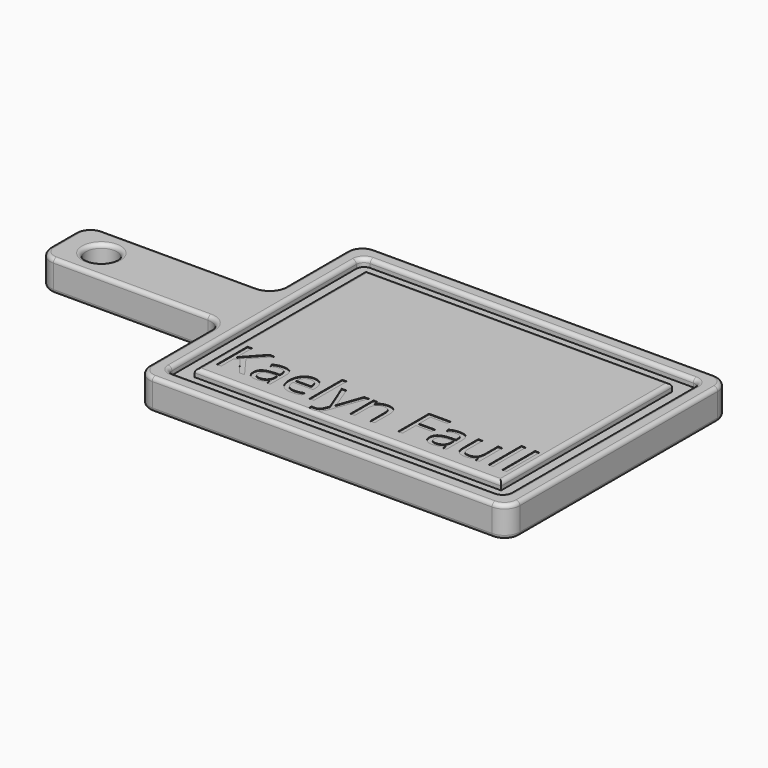
from build123d import *

# Parameters (mm, degrees)
F0_W         = 152.4
F0_H         = 50.8
F1_DEPTH     = 25.4
F2_R         = 12.7
F3_DEPTH     = 25.4
F5_DEPTH     = 6.35
F6_R         = 6.35
F7_R         = 12.7
F8_R         = 3.175
F9_TEXT_SIZE = 44.3979866997
F10_DEPTH    = 0.508


# Not quite as in the source:
# - Text() gives the source's letters only with a copy of the font that has no kerning and outlines rounded to 1/6400 em; it was checked with that copy


with BuildPart() as f1:
    # F0 (on Top) → F1 (new body)
    with BuildSketch(Plane.XY):
        Polygon((0, 88.9), (0, 0), (304.8, 0), (304.8, 228.6), (0, 228.6), (0, 139.7), align=None)
        with Locations((-76.2, 114.3)):
            Rectangle(F0_W, F0_H)
    extrude(amount=F1_DEPTH)

    # F2 (on face) → F3 (cut)
    with BuildSketch(Plane.XY.offset(25.4)):
        with Locations((-120.65, 114.3)):
            Circle(F2_R)
    extrude(amount=-F3_DEPTH, mode=Mode.SUBTRACT)

    # F4 (on face) → F5 (cut)
    with BuildSketch(Plane.XY.offset(25.4)):
        Polygon((13.2080064774, 81.9423422217), (13.2080064774, 13.2080064774), (291.5919935226, 13.2080064774), (291.5919935226, 215.3919935226), (13.2080064774, 215.3919935226), (13.2080064774, 139.7), (13.2080064774, 88.9), align=None)
        Polygon((278.3839935226, 26.4160064774), (26.4160064774, 26.4160064774), (26.4160064774, 82.325167954), (26.4160064774, 88.9), (26.4160064774, 139.7), (26.4160064774, 202.1839935226), (278.3839935226, 202.1839935226), align=None, mode=Mode.SUBTRACT)
    extrude(amount=-F5_DEPTH, mode=Mode.SUBTRACT)

    # F6
    f6_edges = [f1.edges().sort_by_distance(p)[0] for p in [
        (13.208006, 215.391994, 22.225),
        (291.591994, 215.391994, 22.225),
        (291.591994, 13.208006, 22.225),
        (13.208006, 13.208006, 22.225),
    ]]
    fillet(f6_edges, radius=F6_R)

    # F7
    f7_edges = [f1.edges().sort_by_distance(p)[0] for p in [
        (0, 228.6, 12.7),
        (-152.4, 139.7, 12.7),
        (-152.4, 88.9, 12.7),
        (0, 0, 12.7),
        (0, 88.9, 12.7),
        (0, 139.7, 12.7),
        (304.8, 0, 12.7),
        (304.8, 228.6, 12.7),
    ]]
    fillet(f7_edges, radius=F7_R)

    # F8
    f8_edges = [f1.edges().sort_by_distance(p)[0] for p in [
        (278.383994, 114.3, 25.4),
        (152.4, 26.416006, 25.4),
        (26.416006, 114.3, 25.4),
        (152.4, 202.183994, 25.4),
        (0, 44.45, 25.4),
        (-3.719744, 85.180256, 25.4),
        (3.719744, 3.719744, 25.4),
        (-76.2, 88.9, 25.4),
        (152.4, 0, 25.4),
        (-148.680256, 92.619744, 25.4),
        (301.080256, 3.719744, 25.4),
        (-152.4, 114.3, 25.4),
        (304.8, 114.3, 25.4),
        (-148.680256, 135.980256, 25.4),
        (301.080256, 224.880256, 25.4),
        (-76.2, 139.7, 25.4),
        (152.4, 228.6, 25.4),
        (-3.719744, 143.419744, 25.4),
        (3.719744, 224.880256, 25.4),
        (0, 184.15, 25.4),
        (152.4, 13.208006, 25.4),
        (15.067878, 15.067878, 25.4),
        (289.732122, 15.067878, 25.4),
        (13.208006, 114.3, 25.4),
        (291.591994, 114.3, 25.4),
        (15.067878, 213.532122, 25.4),
        (289.732122, 213.532122, 25.4),
        (152.4, 215.391994, 25.4),
        (-133.35, 114.3, 25.4),
        (0, 44.45, 0),
        (-3.719744, 85.180256, 0),
        (3.719744, 3.719744, 0),
        (-76.2, 88.9, 0),
        (152.4, 0, 0),
        (-148.680256, 92.619744, 0),
        (301.080256, 3.719744, 0),
        (-152.4, 114.3, 0),
        (304.8, 114.3, 0),
        (-148.680256, 135.980256, 0),
        (301.080256, 224.880256, 0),
        (-76.2, 139.7, 0),
        (152.4, 228.6, 0),
        (-3.719744, 143.419744, 0),
        (3.719744, 224.880256, 0),
        (0, 184.15, 0),
        (-133.35, 114.3, 0),
    ]]
    fillet(f8_edges, radius=F8_R)

    # F9 (on face) → F10 (cut)
    with BuildSketch(Plane.XY.offset(25.4)):
        with Locations((29.5910064774, 39.6401254587)):
            Text('Kaelyn Faull', F9_TEXT_SIZE, font='Open Sans', text_align=(TextAlign.LEFT, TextAlign.BOTTOM))
    extrude(amount=-F10_DEPTH, mode=Mode.SUBTRACT)


solid = f1.part
